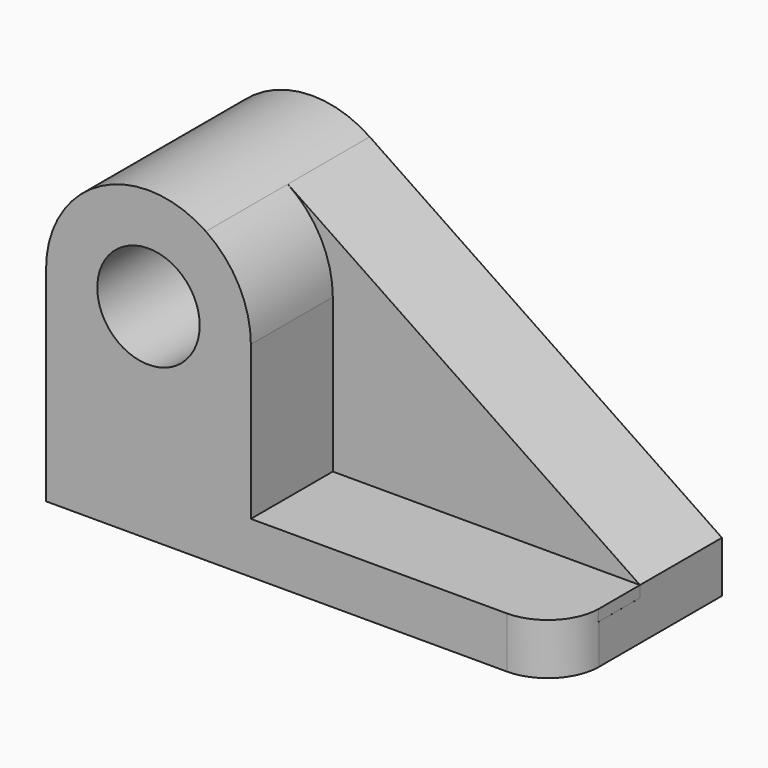
from build123d import *

# Parameters (mm, degrees)
F0_R        = 12.7
F1_DEPTH    = 25.4
F2_R        = 12.7
F3_DEPTH    = 25.4
F4_T1_DEPTH = 73.3820900713
F4_T6_DEPTH = 61.9223878104


# Not quite as in the source:
# - a fillet or chamfer that OpenCascade refuses, or shapes differently, is made with other operations: its cross-section is extruded or revolved along the edge and cut away or added


with BuildPart() as f1:
    # F0 (on Front) → F1 (new body)
    with BuildSketch(Plane.XZ):
        with BuildLine():
            Line((51.8036965728, 2.8171599331), (-35.5584302991, 61.9514882749))
            ThreePointArc((-35.5584302991, 61.9514882749), (-61.7025627589, 63.353759246), (-75.1963034272, 40.9171599331))
            Line((-75.1963034272, 40.9171599331), (-75.1963034272, -9.8828400669))
            Line((-75.1963034272, -9.8828400669), (51.8036965728, -9.8828400669))
            Line((51.8036965728, -9.8828400669), (51.8036965728, 2.8171599331))
        make_face()
        with Locations((-49.7963034272, 40.9171599331)):
            Circle(F0_R, mode=Mode.SUBTRACT)
    extrude(amount=F1_DEPTH)

    # F2 (on face) → F3 (join)
    with BuildSketch(Plane.XZ.offset(25.4)):
        with BuildLine():
            Line((-24.3963034272, 2.8171599331), (-24.3963034272, 40.9171599331))
            ThreePointArc((-24.3963034272, 40.9171599331), (-27.3597041143, 52.8234192648), (-35.5584302991, 61.9514882749))
            ThreePointArc((-35.5584302991, 61.9514882749), (-61.7025627589, 63.353759246), (-75.1963034272, 40.9171599331))
            Line((-75.1963034272, 40.9171599331), (-75.1963034272, 0))
            Line((-75.1963034272, 0), (-75.1963034272, -9.8828400669))
            Line((-75.1963034272, -9.8828400669), (51.8036965728, -9.8828400669))
            Line((51.8036965728, -9.8828400669), (51.8036965728, -0.3670600709))
            Line((51.8036965728, -0.3670600709), (51.8036965728, 0))
            Line((51.8036965728, 0), (51.7987225249, 0))
            Line((51.7987225249, 0), (51.8036965728, 2.8171599331))
            Line((51.8036965728, 2.8171599331), (-24.3963034272, 2.8171599331))
        make_face()
        with Locations((-49.7963034272, 40.9171599331)):
            Circle(F2_R, mode=Mode.SUBTRACT)
    extrude(amount=F3_DEPTH)

    # F4: fillet of radius 12.7 on 2 edges, made by hand

    # F4_s2 → F4_t1 (cut)
    with BuildSketch(Plane.XY.offset(-41.6324650691)):
        with BuildLine():
            ThreePointArc((39.1038465728, -50.80015), (48.0841026938, -47.0804061211), (51.8038465728, -38.10015))
            Line((51.8038465728, -38.10015), (52.0578465728, -38.10015))
            ThreePointArc((52.0578465728, -38.10015), (52.0576965728, -44.450075), (52.0576965728, -50.8))
            Line((52.0576965728, -50.8), (51.8036965728, -51.054))
            ThreePointArc((51.8036965728, -51.054), (45.4537715728, -51.054), (39.1038465728, -51.05415))
            Line((39.1038465728, -51.05415), (39.1038465728, -50.80015))
        make_face()
    extrude(amount=F4_T1_DEPTH, mode=Mode.SUBTRACT)


with BuildPart() as f4_tool4:
    # F4_s5 → F4_t6 (new body)
    with BuildSketch(Plane.YZ.offset(82.762403454)):
        with BuildLine():
            ThreePointArc((-50.8001462633, -9.8828067947), (-46.3384346707, -2.7734597017), (-38.4165172484, 0.00015))
            Line((-38.4165172484, 0.00015), (-38.4165172484, 0.25415))
            ThreePointArc((-38.4165172484, 0.25415), (-44.6082586242, 0.254), (-50.8, 0.254))
            Line((-50.8, 0.254), (-51.054, 0))
            ThreePointArc((-51.054, 0), (-51.054, -4.9414033973), (-51.0478188436, -9.8264659306))
            Line((-51.0478188436, -9.8264659306), (-50.8001462633, -9.8828067947))
        make_face()
    extrude(amount=-F4_T6_DEPTH)

    split(bisect_by=Plane(origin=(51.7985610464, 0, -0.0914568329), x_dir=(0, 1, 0), z_dir=(0.9999984413, 0, -0.0017656222)), keep=Keep.TOP)


with BuildPart() as f1_1:
    add(f1.part)

    # F4_t3: cut F4_tool4
    add(f4_tool4.part, mode=Mode.SUBTRACT)


solid = f1_1.part
